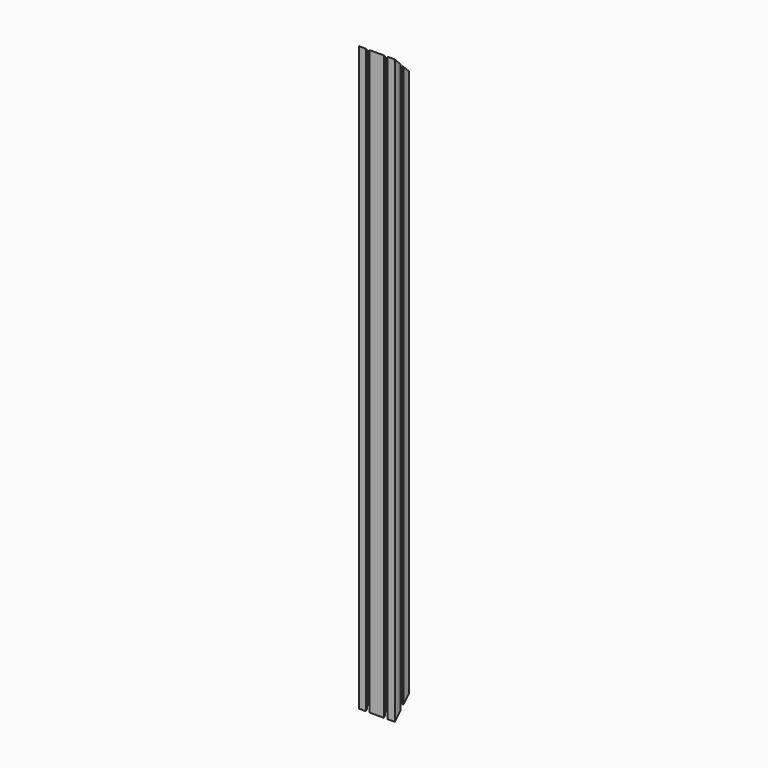
from build123d import *

# Parameters (mm, degrees)
F0_R     = 3
F0_R_2   = 2.5
F1_DEPTH = 973
F2_R     = 2
F3_R     = 7
F5_DEPTH = 30


# Not quite as in the source:
# - a feature names something its author has since deleted; it is built from what else it names


with BuildPart() as f1:
    # F0 (on Top) → F1 (new body)
    with BuildSketch(Plane.XY):
        with BuildLine():
            Line((18.15, -15), (30, -15))
            Line((30, -15), (30, -3.15))
            Line((30, -3.15), (27.5, -3.15))
            Line((27.5, -3.15), (27.5, -5.15))
            Line((27.5, -5.15), (21.5477069044, -5.15))
            ThreePointArc((21.5477069044, -5.15), (19.5, 0), (21.5477069044, 5.15))
            Line((21.5477069044, 5.15), (27.5, 5.15))
            Line((27.5, 5.15), (27.5, 3.15))
            Line((27.5, 3.15), (30, 3.15))
            Line((30, 3.15), (30, 15))
            Line((30, 15), (18.15, 15))
            Line((18.15, 15), (18.15, 12.5))
            Line((18.15, 12.5), (20.15, 12.5))
            Line((20.15, 12.5), (20.15, 6.5477069044))
            ThreePointArc((20.15, 6.5477069044), (15, 4.5), (9.85, 6.5477069044))
            Line((9.85, 6.5477069044), (9.85, 12.5))
            Line((9.85, 12.5), (11.85, 12.5))
            Line((11.85, 12.5), (11.85, 15))
            Line((11.85, 15), (-11.85, 15))
            Line((-11.85, 15), (-11.85, 12.5))
            Line((-11.85, 12.5), (-9.85, 12.5))
            Line((-9.85, 12.5), (-9.85, 6.5477069044))
            ThreePointArc((-9.85, 6.5477069044), (-15, 4.5), (-20.15, 6.5477069044))
            Line((-20.15, 6.5477069044), (-20.15, 12.5))
            Line((-20.15, 12.5), (-18.15, 12.5))
            Line((-18.15, 12.5), (-18.15, 15))
            Line((-18.15, 15), (-30, 15))
            Line((-30, 15), (-30, 3.15))
            Line((-30, 3.15), (-27.5, 3.15))
            Line((-27.5, 3.15), (-27.5, 5.15))
            Line((-27.5, 5.15), (-21.5477069044, 5.15))
            ThreePointArc((-21.5477069044, 5.15), (-19.5, 0), (-21.5477069044, -5.15))
            Line((-21.5477069044, -5.15), (-27.5, -5.15))
            Line((-27.5, -5.15), (-27.5, -3.15))
            Line((-27.5, -3.15), (-30, -3.15))
            Line((-30, -3.15), (-30, -15))
            Line((-30, -15), (-18.15, -15))
            Line((-18.15, -15), (-18.15, -12.5))
            Line((-18.15, -12.5), (-20.15, -12.5))
            Line((-20.15, -12.5), (-20.15, -6.5477069044))
            ThreePointArc((-20.15, -6.5477069044), (-15, -4.5), (-9.85, -6.5477069044))
            Line((-9.85, -6.5477069044), (-9.85, -12.5))
            Line((-9.85, -12.5), (-11.85, -12.5))
            Line((-11.85, -12.5), (-11.85, -15))
            Line((-11.85, -15), (11.85, -15))
            Line((11.85, -15), (11.85, -12.5))
            Line((11.85, -12.5), (9.85, -12.5))
            Line((9.85, -12.5), (9.85, -6.5477069044))
            ThreePointArc((9.85, -6.5477069044), (15, -4.5), (20.15, -6.5477069044))
            Line((20.15, -6.5477069044), (20.15, -12.5))
            Line((20.15, -12.5), (18.15, -12.5))
            Line((18.15, -12.5), (18.15, -15))
        make_face()
        with Locations((-25, -10)):
            Circle(F0_R, mode=Mode.SUBTRACT)
        with Locations((25, -10)):
            Circle(F0_R, mode=Mode.SUBTRACT)
        with Locations((-15, 0)):
            Circle(F0_R_2, mode=Mode.SUBTRACT)
        with Locations((-25, 10)):
            Circle(F0_R, mode=Mode.SUBTRACT)
        Polygon((-7, 7), (-7, 12.5), (0, 12.5), (7, 12.5), (7, 7), (10, 0), (7, -7), (7, -12.5), (0, -12.5), (-7, -12.5), (-7, -7), (-10, 0), align=None, mode=Mode.SUBTRACT)
        with Locations((15, 0)):
            Circle(F0_R_2, mode=Mode.SUBTRACT)
        with Locations((25, 10)):
            Circle(F0_R, mode=Mode.SUBTRACT)
    extrude(amount=F1_DEPTH)

    # F2
    f2_edges = [f1.edges().sort_by_distance(p)[0] for p in [
        (-7, 12.5, 486.5),
        (7, 12.5, 486.5),
    ]]
    fillet(f2_edges, radius=F2_R)

    # F3
    f3_edges = [f1.edges().sort_by_distance(p)[0] for p in [
        (-7, 7, 486.5),
        (-10, 0, 486.5),
        (7, 7, 486.5),
        (10, 0, 486.5),
    ]]
    fillet(f3_edges, radius=F3_R)

    # F4 (on Right) → F5 (cut, symmetric)
    with BuildSketch(Plane.YZ):
        Polygon((15, 30), (-15, 0), (15, 0), align=None)
        Polygon((15, 973), (-15, 973), (15, 943), align=None)
    extrude(amount=F5_DEPTH, both=True, mode=Mode.SUBTRACT)


solid = f1.part
